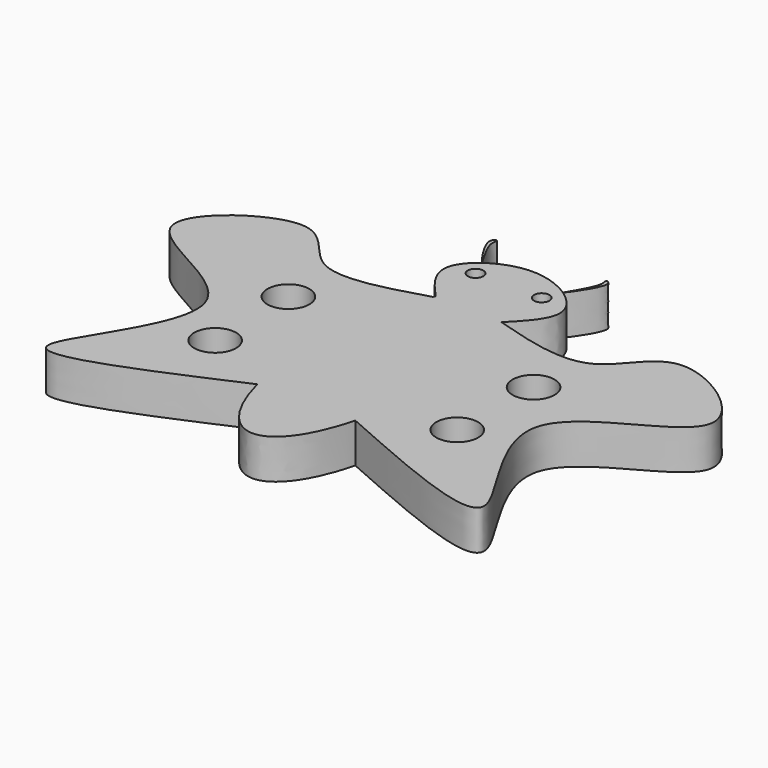
from build123d import *

# Parameters (mm, degrees)
F0_R     = 4.4252747669
F0_R_2   = 4.4252734516
F0_R_3   = 1.6403995765
F1_DEPTH = 8.382


with BuildPart() as f1:
    # F0 (on Top) → F1 (new body)
    with BuildSketch(Plane.XY):
        with BuildLine():
            add(Edge.make_bspline(
                [(-10.3449848816, -17.0957947478), (-6.6871748873, -31.254376115), (0, -31.254376115)],
                knots=[5.2911520049, 5.2911520049, 5.2911520049, 6.2831853072, 6.2831853072, 6.2831853072], degree=2, weights=[1, 0.8794853137, 1]))
            add(Edge.make_bspline(
                [(0, -31.254376115), (6.6871748873, -31.254376115), (10.3449848816, -17.0957947478)],
                knots=[0, 0, 0, 0.9920333023, 0.9920333023, 0.9920333023], degree=2, weights=[1, 0.8794853137, 1]))
            add(Edge.make_bspline(
                [(10.3449848816, -17.0957947478), (16.8015802945, 7.8962719953), (7.2261885702, 25.3537539647)],
                knots=[0.9920333023, 0.9920333023, 0.9920333023, 2.5170087891, 2.5170087891, 2.5170087891], degree=2, weights=[1, 0.7231199098, 1]))
            add(Edge.make_bspline(
                [(7.2261885702, 25.3537539647), (0.1789018258, 38.2020932092), (-6.9867295528, 25.7795179286)],
                knots=[2.5170087891, 2.5170087891, 2.5170087891, 3.7424891768, 3.7424891768, 3.7424891768], degree=2, weights=[1, 0.8180751747, 1]))
            add(Edge.make_bspline(
                [(-6.9867295528, 25.7795179286), (-7.1074559957, 25.5702225789), (-7.2261885702, 25.3537539647)],
                knots=[3.7424891768, 3.7424891768, 3.7424891768, 3.7661765181, 3.7661765181, 3.7661765181], degree=2, weights=[1, 0.9999298646, 1]))
            add(Edge.make_bspline(
                [(-7.2261885702, 25.3537539647), (-16.8015802945, 7.8962719953), (-10.3449848816, -17.0957947478)],
                knots=[3.7661765181, 3.7661765181, 3.7661765181, 5.2911520049, 5.2911520049, 5.2911520049], degree=2, weights=[1, 0.7231199098, 1]))
        make_face()
        with BuildLine():
            add(Edge.make_bspline(
                [(10.3449848816, -17.0957947478), (16.8015802945, 7.8962719953), (7.2261885702, 25.3537539647)],
                knots=[0.9920333023, 0.9920333023, 0.9920333023, 2.5170087891, 2.5170087891, 2.5170087891], degree=2, weights=[1, 0.7231199098, 1]))
            add(Edge.make_bspline(
                [(7.2261885702, 25.3537539647), (15.3921379331, 22.8983923283), (30.2097479394, 18.4429941525), (37.0684976545, 38.8295733005), (71.0550420387, 15.0469727271), (19.3838313003, 5.2699497804), (61.4826642588, -39.7069869104), (27.9992409806, -24.9027501664), (10.3449848816, -17.0957947478)],
                knots=[0, 0, 0, 0, 0.1546484689, 0.2805906562, 0.4353572687, 0.6136876134, 0.7961926108, 1, 1, 1, 1], degree=3))
        make_face()
        with Locations((25.5555752665, -9.2021031305)):
            Circle(F0_R, mode=Mode.SUBTRACT)
        with Locations((25.8845034987, 10.5335758999)):
            Circle(F0_R_2, mode=Mode.SUBTRACT)
        with BuildLine():
            add(Edge.make_bspline(
                [(-7.2261885702, 25.3537539647), (-15.3921379331, 22.8983923283), (-30.2097479394, 18.4429941525), (-37.0684976545, 38.8295733005), (-71.0550420387, 15.0469727271), (-19.3838313003, 5.2699497804), (-61.4826642588, -39.7069869104), (-27.9992409806, -24.9027501664), (-10.3449848816, -17.0957947478)],
                knots=[0, 0, 0, 0, 0.1546484689, 0.2805906562, 0.4353572687, 0.6136876134, 0.7961926108, 1, 1, 1, 1], degree=3))
            add(Edge.make_bspline(
                [(-7.2261885702, 25.3537539647), (-16.8015802945, 7.8962719953), (-10.3449848816, -17.0957947478)],
                knots=[3.7661765181, 3.7661765181, 3.7661765181, 5.2911520049, 5.2911520049, 5.2911520049], degree=2, weights=[1, 0.7231199098, 1]))
        make_face()
        with Locations((-25.5555752665, -9.2021031305)):
            Circle(F0_R, mode=Mode.SUBTRACT)
        with Locations((-25.8845034987, 10.5335758999)):
            Circle(F0_R_2, mode=Mode.SUBTRACT)
        with BuildLine():
            add(Edge.make_bspline(
                [(7.2261885702, 25.3537539647), (0.1789018258, 38.2020932092), (-6.9867295528, 25.7795179286)],
                knots=[2.5170087891, 2.5170087891, 2.5170087891, 3.7424891768, 3.7424891768, 3.7424891768], degree=2, weights=[1, 0.8180751747, 1]))
            add(Edge.make_bspline(
                [(8.5713136766, 39.9259235175), (10.7354060152, 38.4602110732), (15.1038018809, 33.2306868528), (10.2124236639, 28.4221517284), (7.2261885702, 25.3537539647)],
                knots=[0.6380001492, 0.6380001492, 0.6380001492, 0.6380001492, 0.7675261923, 1, 1, 1, 1], degree=3))
            add(Edge.make_bspline(
                [(8.5119795385, 39.8723508154), (8.5229433457, 39.8777863957), (8.5430453911, 39.8960024418), (8.5713136766, 39.9259235175)],
                knots=[0, 0, 0, 0, 0.0183737229, 0.0183737229, 0.0183737229, 0.0183737229], degree=3))
            add(Edge.make_bspline(
                [(8.5319371078, 39.9525033879), (8.5013045818, 39.8914829435), (8.4931149026, 39.8629982026), (8.5119795385, 39.8723508154)],
                knots=[0.9683856543, 0.9683856543, 0.9683856543, 0.9683856543, 1, 1, 1, 1], degree=3))
            add(Edge.make_bspline(
                [(-8.5021044631, 39.8795855803), (-6.2350667333, 41.5388744473), (-0.1510298779, 43.8128407788), (6.1498583381, 41.5550580805), (8.5319371078, 39.9525033879)],
                knots=[0.3485096115, 0.3485096115, 0.3485096115, 0.3485096115, 0.4951193448, 0.6372158719, 0.6372158719, 0.6372158719, 0.6372158719], degree=3))
            add(Edge.make_bspline(
                [(-8.5021044631, 39.8795855803), (-8.5010527656, 39.87104658), (-8.5042382353, 39.8685128717), (-8.5119795385, 39.8723508154)],
                knots=[0.9870267184, 0.9870267184, 0.9870267184, 0.9870267184, 1, 1, 1, 1], degree=3))
            add(Edge.make_bspline(
                [(-6.9867295528, 25.7795179286), (-9.8210308405, 28.8941310268), (-14.1395216035, 33.6306798593), (-10.3321105693, 38.5375777726), (-8.5119795385, 39.8723508154)],
                knots=[0, 0, 0, 0, 0.2304641265, 0.3482966249, 0.3482966249, 0.3482966249, 0.3482966249], degree=3))
        make_face()
        with Locations((-6.9867295528, 36.3017208874)):
            Circle(F0_R_3, mode=Mode.SUBTRACT)
        with Locations((6.9867295528, 36.3017208874)):
            Circle(F0_R_3, mode=Mode.SUBTRACT)
        with BuildLine():
            add(Edge.make_bspline(
                [(8.5119795385, 39.8723508154), (8.5229433457, 39.8777863957), (8.5430453911, 39.8960024418), (8.5713136766, 39.9259235175)],
                knots=[0, 0, 0, 0, 0.0183737229, 0.0183737229, 0.0183737229, 0.0183737229], degree=3))
            add(Edge.make_bspline(
                [(8.5319371078, 39.9525033879), (8.5450845804, 39.9436583639), (8.5582101466, 39.9347983731), (8.5713136766, 39.9259235175)],
                knots=[0.6372158719, 0.6372158719, 0.6372158719, 0.6372158719, 0.6380001492, 0.6380001492, 0.6380001492, 0.6380001492], degree=3))
            add(Edge.make_bspline(
                [(8.5319371078, 39.9525033879), (8.5013045818, 39.8914829435), (8.4931149026, 39.8629982026), (8.5119795385, 39.8723508154)],
                knots=[0.9683856543, 0.9683856543, 0.9683856543, 0.9683856543, 1, 1, 1, 1], degree=3))
        make_face()
        with BuildLine():
            add(Edge.make_bspline(
                [(8.5319371078, 39.9525033879), (8.5450845804, 39.9436583639), (8.5582101466, 39.9347983731), (8.5713136766, 39.9259235175)],
                knots=[0.6372158719, 0.6372158719, 0.6372158719, 0.6372158719, 0.6380001492, 0.6380001492, 0.6380001492, 0.6380001492], degree=3))
            add(Edge.make_bspline(
                [(8.5713136766, 39.9259235175), (9.0990120583, 40.4844753685), (13.836582329, 46.9972267895), (10.9898921098, 48.0170311383), (12.470083688, 46.0671885777), (8.8258981265, 40.5380780796), (8.5319371078, 39.9525033879)],
                knots=[0.0183737229, 0.0183737229, 0.0183737229, 0.0183737229, 0.3613653002, 0.5000627444, 0.6650027319, 0.9683856543, 0.9683856543, 0.9683856543, 0.9683856543], degree=3))
        make_face()
        with BuildLine():
            add(Edge.make_bspline(
                [(-8.5119795385, 39.8723508154), (-8.7276102802, 39.9792551226), (-13.9174699733, 46.9682494281), (-10.9898921098, 48.0170311383), (-12.5155390766, 46.0073106183), (-8.528209793, 40.0915414305), (-8.5021044631, 39.8795855803)],
                knots=[0, 0, 0, 0, 0.3613653002, 0.5000627444, 0.6650027319, 0.9870267184, 0.9870267184, 0.9870267184, 0.9870267184], degree=3))
            add(Edge.make_bspline(
                [(-8.5119795385, 39.8723508154), (-8.5086895842, 39.8747634671), (-8.5053978916, 39.8771750561), (-8.5021044631, 39.8795855803)],
                knots=[0.3482966249, 0.3482966249, 0.3482966249, 0.3482966249, 0.3485096115, 0.3485096115, 0.3485096115, 0.3485096115], degree=3))
        make_face()
        with BuildLine():
            add(Edge.make_bspline(
                [(-8.5119795385, 39.8723508154), (-8.5086895842, 39.8747634671), (-8.5053978916, 39.8771750561), (-8.5021044631, 39.8795855803)],
                knots=[0.3482966249, 0.3482966249, 0.3482966249, 0.3482966249, 0.3485096115, 0.3485096115, 0.3485096115, 0.3485096115], degree=3))
            add(Edge.make_bspline(
                [(-8.5021044631, 39.8795855803), (-8.5010527656, 39.87104658), (-8.5042382353, 39.8685128717), (-8.5119795385, 39.8723508154)],
                knots=[0.9870267184, 0.9870267184, 0.9870267184, 0.9870267184, 1, 1, 1, 1], degree=3))
        make_face()
    extrude(amount=F1_DEPTH)


solid = f1.part
